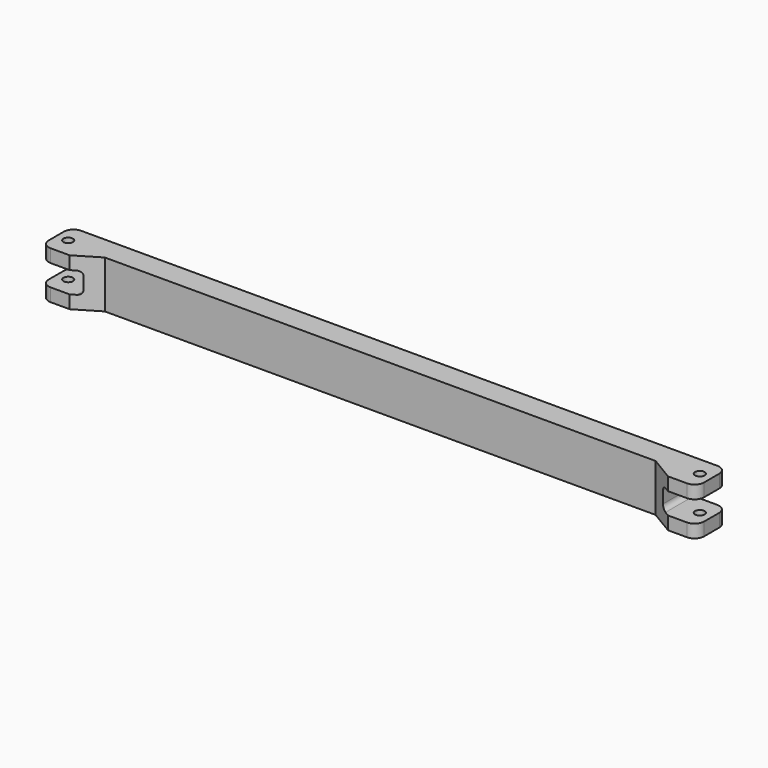
from build123d import *

# Parameters (mm, degrees)
F1_DEPTH      = 4
F2_R          = 1
F3_DEPTH      = 5.001
F3_DEPTH_BACK = 5.001
F4_W          = 126
F4_H          = 10
F5_DEPTH      = 10
F6_SIZE2      = 2.99999
F6_SIZE       = 4.99999
F7_R          = 2
F8_R          = 1


# Not quite as in the source:
# - a fillet or chamfer is up to 0.001 mm smaller than in the source, because OpenCascade refuses the exact size


with BuildPart() as f1:
    # F0 (on Front) → F1 (new body, symmetric)
    with BuildSketch(Plane.XZ):
        Polygon((69, 2.25), (69, 5), (-69, 5), (-69, 2.25), (-61, 2.25), (-61, -2.25), (-69, -2.25), (-69, -5), (69, -5), (69, -2.25), (61, -2.25), (61, 2.25), align=None)
    extrude(amount=F1_DEPTH, both=True)

    # F2 (on Top) → F3 (cut, two sides)
    with BuildSketch(Plane.XY) as f3_sk:
        with Locations((-66.5, 0)):
            Circle(F2_R)
        with Locations((66.5, 0)):
            Circle(F2_R)
    extrude(amount=-F3_DEPTH, mode=Mode.SUBTRACT)
    extrude(f3_sk.sketch, amount=F3_DEPTH_BACK, mode=Mode.SUBTRACT)

    # F4 (on Top) → F5 (cut, symmetric)
    with BuildSketch(Plane.XY):
        with Locations((0, -6)):
            Rectangle(F4_W, F4_H)
    extrude(amount=F5_DEPTH, both=True, mode=Mode.SUBTRACT)

    # F6 (size 5 and 3 in the source; OpenCascade refuses exactly that, so slightly less here)
    f6_edges = [f1.edges().sort_by_distance(p)[0] for p in [
        (-63, -1, 3.625),
        (63, -1, 3.625),
    ]]
    f6_side = f1.faces().sort_by_distance((0, -1, 0))[0]
    chamfer(f6_edges, length=F6_SIZE, length2=F6_SIZE2, reference=f6_side)

    # F7
    f7_edges = [f1.edges().sort_by_distance(p)[0] for p in [
        (-69, 4, 3.625),
        (-69, 4, -3.625),
        (-69, -4, 3.625),
        (-69, -4, -3.625),
        (69, -4, 3.625),
        (69, -4, -3.625),
        (69, 4, -3.625),
        (69, 4, 3.625),
    ]]
    fillet(f7_edges, radius=F7_R)

    # F8
    f8_edges = [f1.edges().sort_by_distance(p)[0] for p in [
        (61, 0.600004, -2.25),
        (61, 0.600004, 2.25),
        (-61, 0.600004, 2.25),
        (-61, 0.600004, -2.25),
    ]]
    fillet(f8_edges, radius=F8_R)


solid = f1.part
